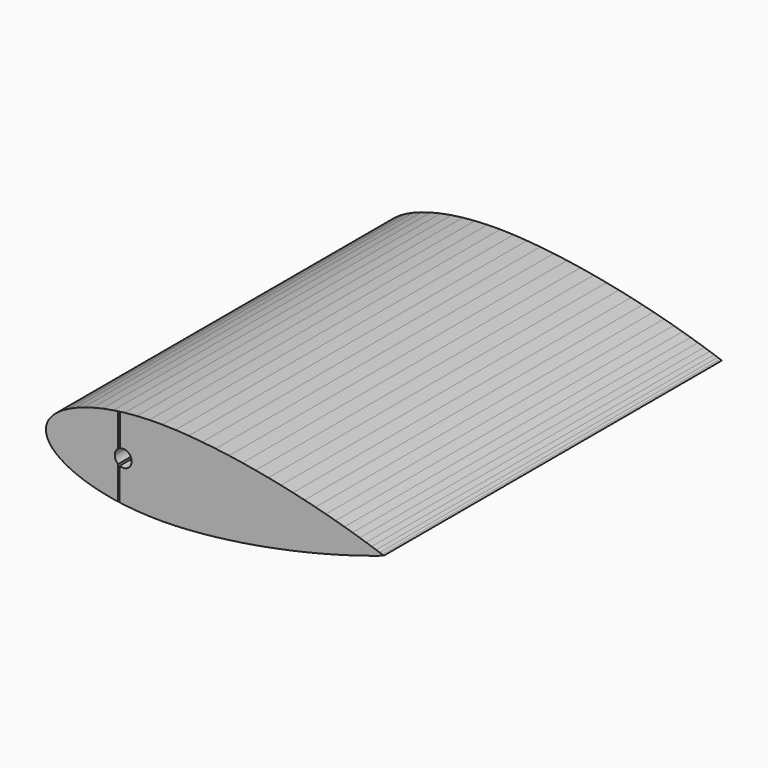
from build123d import *

# Parameters (mm, degrees)
F1_DEPTH = 1000
F3_DEPTH = 1000
F4_DEPTH = 1100


# Not quite as in the source:
# - a feature names something its author has since deleted; it is built from what else it names


with BuildPart() as f1:
    # F0 (on Front) → F1 (new body)
    with BuildSketch(Plane.XZ):
        Polygon((398.8592052974, -22.0067325898), (399.1788252872, -21.8985260996), (398.86, -21.788), (395.252, -20.532), (389.268, -18.468), (380.924, -15.636), (370.284, -12.092), (357.388, -7.884), (342.308, -3.092), (325.124, 2.196), (305.94, 7.9), (284.86, 13.924), (261.996, 20.188), (237.476, 26.58), (211.46, 33.028), (184.092, 39.412), (155.54, 45.66), (125.964, 51.676), (95.556, 57.364), (64.508, 62.644), (32.996, 67.412), (1.236, 71.604), (-30.58, 75.124), (-62.236, 77.908), (-93.804, 79.86), (-125.172, 80.74), (-155.748, 80.484), (-185.332, 79.076), (-213.692, 76.532), (-240.636, 72.9), (-265.956, 68.236), (-289.484, 62.612), (-311.052, 56.124), (-330.516, 48.892), (-347.748, 41.02), (-362.66, 32.636), (-375.156, 23.868), (-385.18, 14.828), (-392.684, 5.62), (-397.644, -3.66), (-400.06, -12.948), (-399.9816032326, -18.9950039949), (-400.1039374883, -25.0412786908), (-397.7554909925, -34.3465889519), (-392.863053528, -43.6623849811), (-385.4261600494, -52.9246684677), (-375.4681123548, -62.0372675544), (-363.0361534783, -70.8958362025), (-348.1854681119, -79.3879704541), (-331.0111236302, -87.3849761202), (-311.6001876192, -94.7582171427), (-290.0799010007, -101.4027661761), (-266.5933880129, -107.1975800363), (-241.3079466524, -112.0454405133), (-214.3910493078, -115.8731287637), (-186.0502835732, -118.6231348681), (-156.4772955956, -120.2460649573), (-125.9039629887, -120.7242336641), (-94.530396734, -120.0721872989), (-62.949046248, -118.3496225018), (-31.2736524944, -115.7957191071), (0.567085058, -112.5069977565), (32.356707066, -108.5458872321), (63.9025210304, -104.006989863), (94.988067608, -98.9527344313), (125.4365957465, -93.4858393163), (155.0555292079, -87.6849072697), (183.6521754929, -81.6445406207), (211.0658412572, -75.4595742212), (237.1280077599, -69.2007854261), (261.6938068426, -62.9871247152), (284.602719553, -56.8894275739), (305.7259354409, -51.0187609546), (324.9508761562, -45.4543089157), (342.1728468763, -40.2913132239), (357.2872690402, -35.6090160683), (370.2135053222, -31.494833819), (380.8789763165, -28.0282411878), (389.2433342948, -25.256946254), (395.2421740321, -23.2364824938), align=None)
    extrude(amount=F1_DEPTH)

    # F2 (on face) → F3 (cut)
    with BuildSketch(Plane.XZ.offset(1000)):
        with BuildLine():
            ThreePointArc((-229.6033561446, -3.6511614936), (-235.4817946773, -10.6760485755), (-237.6118033553, -19.5849284785))
            Line((-237.6118033553, -19.5849284785), (-197.6120673578, -19.7302561417))
            ThreePointArc((-197.6120673578, -19.7302561417), (-206.6231942764, -2.9468900665), (-225.6033561446, -1.3235476449))
            Line((-225.6033561446, -1.3235476449), (-225.6033561446, 73.9173274625))
            Line((-225.6033561446, 73.9173274625), (-229.6033561446, 73.3781350635))
            Line((-229.6033561446, 73.3781350635), (-229.6033561446, -3.6511614936))
        make_face()
        with BuildLine():
            Line((-197.6120673578, -19.7302561417), (-237.6118033553, -19.5849284785))
            ThreePointArc((-237.6118033553, -19.5849284785), (-235.5465858175, -28.5090505427), (-229.7193476609, -35.5764668712))
            ThreePointArc((-229.7193476609, -35.5764668712), (-227.7962509426, -36.8703700071), (-225.736366484, -37.9330846114))
            ThreePointArc((-225.736366484, -37.9330846114), (-206.744909945, -36.4477012646), (-197.6120673578, -19.7302561417))
        make_face()
        with BuildLine():
            ThreePointArc((-225.736366484, -37.9330846114), (-227.7962509426, -36.8703700071), (-229.7193476609, -35.5764668712))
            Line((-229.7193476609, -35.5764668712), (-230.2790683503, -112.6037298424))
            Line((-230.2790683503, -112.6037298424), (-226.2830919036, -113.1719733475))
            Line((-226.2830919036, -113.1719733475), (-225.736366484, -37.9330846114))
        make_face()
    extrude(amount=-F3_DEPTH, mode=Mode.SUBTRACT)

    # F2 (on face) → F4 (cut)
    with BuildSketch(Plane.XZ.offset(1000)):
        with BuildLine():
            ThreePointArc((-229.6033561446, -3.6511614936), (-235.4817946773, -10.6760485755), (-237.6118033553, -19.5849284785))
            Line((-237.6118033553, -19.5849284785), (-197.6120673578, -19.7302561417))
            ThreePointArc((-197.6120673578, -19.7302561417), (-206.6231942764, -2.9468900665), (-225.6033561446, -1.3235476449))
            Line((-225.6033561446, -1.3235476449), (-225.6033561446, 73.9173274625))
            Line((-225.6033561446, 73.9173274625), (-229.6033561446, 73.3781350635))
            Line((-229.6033561446, 73.3781350635), (-229.6033561446, -3.6511614936))
        make_face()
        with BuildLine():
            Line((-197.6120673578, -19.7302561417), (-237.6118033553, -19.5849284785))
            ThreePointArc((-237.6118033553, -19.5849284785), (-235.5465858175, -28.5090505427), (-229.7193476609, -35.5764668712))
            ThreePointArc((-229.7193476609, -35.5764668712), (-227.7962509426, -36.8703700071), (-225.736366484, -37.9330846114))
            ThreePointArc((-225.736366484, -37.9330846114), (-206.744909945, -36.4477012646), (-197.6120673578, -19.7302561417))
        make_face()
        with BuildLine():
            ThreePointArc((-225.736366484, -37.9330846114), (-227.7962509426, -36.8703700071), (-229.7193476609, -35.5764668712))
            Line((-229.7193476609, -35.5764668712), (-230.2790683503, -112.6037298424))
            Line((-230.2790683503, -112.6037298424), (-226.2830919036, -113.1719733475))
            Line((-226.2830919036, -113.1719733475), (-225.736366484, -37.9330846114))
        make_face()
    extrude(amount=-F4_DEPTH, mode=Mode.SUBTRACT)


solid = f1.part
